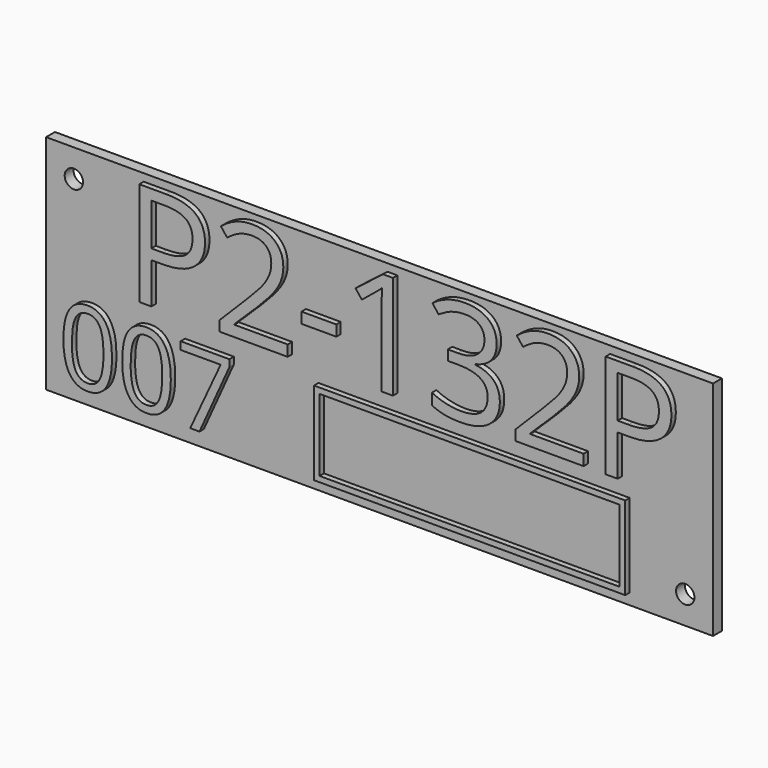
from build123d import *

# Parameters (mm, degrees)
F0_W         = 120
F0_H         = 40
F1_DEPTH     = 2
F3_D         = 3.3
F4_TEXT_SIZE = 26.1352499183
F5_DEPTH     = 1
F6_TEXT_SIZE = 18.5054667028
F7_DEPTH     = 1
F8_W         = 56
F8_H         = 15
F8_W_2       = 53.99999962
F8_H_2       = 12.99999962
F9_DEPTH     = 1


# Not quite as in the source:
# - Text() gives the source's letters only with a copy of the font that has no kerning and outlines rounded to 1/6400 em; it was checked with that copy


with BuildPart() as f1:
    # F0 (on Front) → F1 (new body)
    with BuildSketch(Plane.XZ):
        Rectangle(F0_W, F0_H)
    extrude(amount=F1_DEPTH)

    # F3 (through all)
    with Locations(Plane.XZ.offset(2)):
        with Locations((-55, 15), (55, -15)):
            Hole(F3_D / 2)

    # F4 (on face) → F5 (join)
    with BuildSketch(Plane.XZ.offset(2)):
        with Locations((-45, 0)):
            Text('P2-132P', F4_TEXT_SIZE, font='Open Sans', text_align=(TextAlign.LEFT, TextAlign.BOTTOM))
    extrude(amount=F5_DEPTH)

    # F6 (on face) → F7 (join)
    with BuildSketch(Plane.XZ.offset(2)):
        with Locations((-57, -17)):
            Text('007', F6_TEXT_SIZE, font='Open Sans', text_align=(TextAlign.LEFT, TextAlign.BOTTOM))
    extrude(amount=F7_DEPTH)

    # F8 (on face) → F9 (join)
    with BuildSketch(Plane.XZ.offset(2)):
        with Locations((17, -10.5)):
            Rectangle(F8_W, F8_H)
        with Locations((17, -10.5)):
            Rectangle(F8_W_2, F8_H_2, mode=Mode.SUBTRACT)
    extrude(amount=F9_DEPTH)


solid = f1.part
